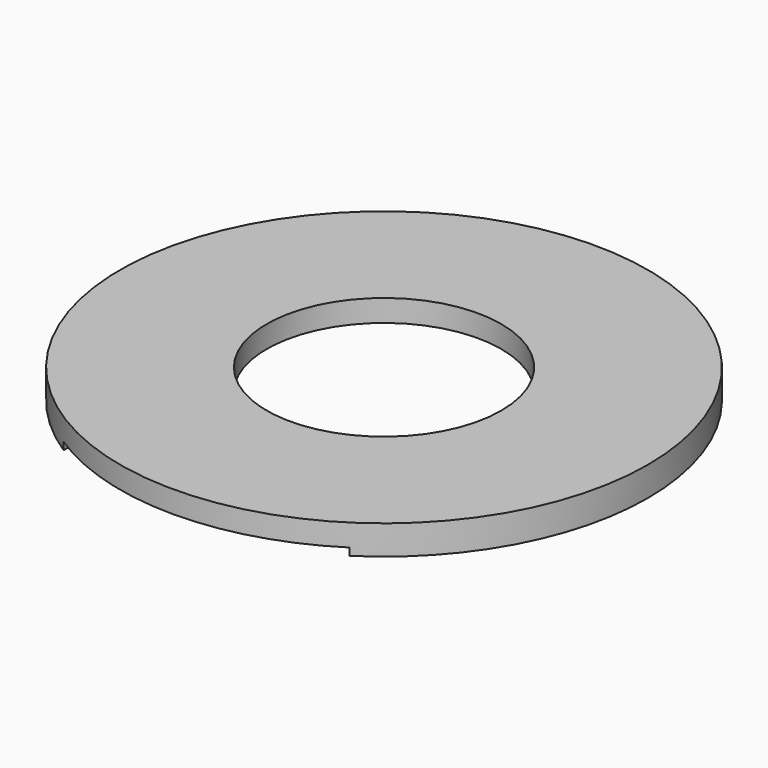
from build123d import *

# Parameters (mm, degrees)
F0_R     = 9
F0_R_2   = 4
F1_DEPTH = 1
F2_R     = 4
F3_DEPTH = 0.25


with BuildPart() as f1:
    # F0 (on Top) → F1 (new body)
    with BuildSketch(Plane.XY):
        Circle(F0_R)
        Circle(F0_R_2, mode=Mode.SUBTRACT)
    extrude(amount=F1_DEPTH)

    # F2 (on face) → F3 (cut)
    with BuildSketch(Plane(origin=(0, 0, 0), x_dir=(1, 0, 0), z_dir=(0, 0, -1))):
        with BuildLine():
            ThreePointArc((4.875, 7.5653403757), (2.5408597579, 8.6338885614), (0, 9))
            ThreePointArc((0, 9), (-2.5408597579, 8.6338885614), (-4.875, 7.5653403757))
            Line((-4.875, 7.5653403757), (-4.875, -7.5653403757))
            ThreePointArc((-4.875, -7.5653403757), (-2.5408597579, -8.6338885614), (0, -9))
            ThreePointArc((0, -9), (2.5408597579, -8.6338885614), (4.875, -7.5653403757))
            Line((4.875, -7.5653403757), (4.875, 7.5653403757))
        make_face()
        Circle(F2_R, mode=Mode.SUBTRACT)
        Circle(F2_R)
    extrude(amount=-F3_DEPTH, mode=Mode.SUBTRACT)


solid = f1.part
